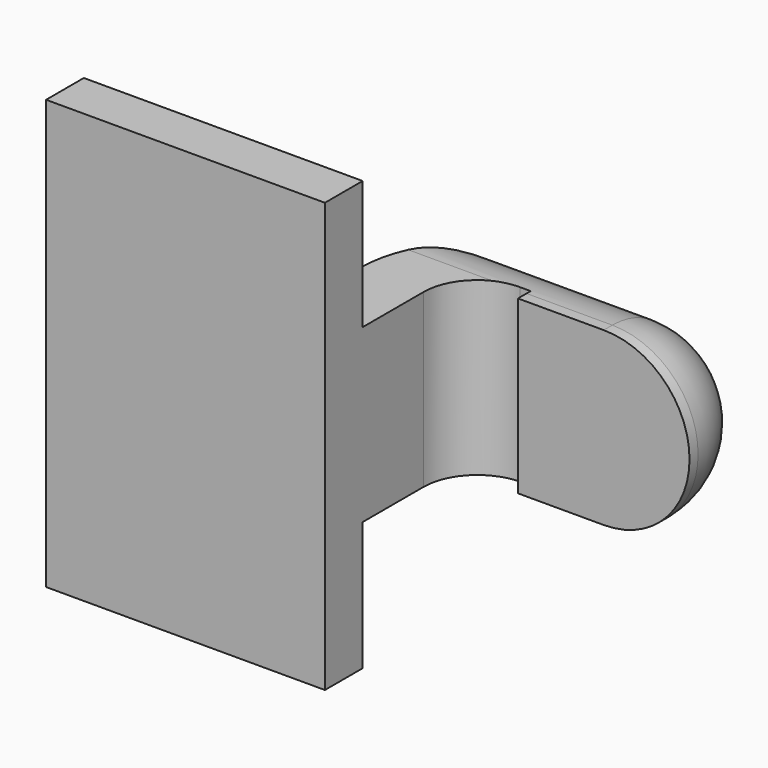
from build123d import *

# Parameters (mm, degrees)
F1_DEPTH    = 63.5
F0_W        = 25.4
F0_H        = 19.05
F0_H_2      = 4.7752
F0_H_3      = 4.7498
F2_DEPTH    = 25.4
F3_DEPTH    = 3.175
F5_T1_DEPTH = 88.9
F5_T4_ANGLE = 180
F6_SIZE     = 5.08


# Not quite as in the source:
# - a fillet or chamfer that OpenCascade refuses, or shapes differently, is made with other operations: its cross-section is extruded or revolved along the edge and cut away or added


with BuildPart() as f1:
    # F0 (on Top) → F1 (new body, symmetric)
    with BuildSketch(Plane.XY):
        Polygon((41.275, -9.525), (41.275, 9.525), (22.225, 9.525), (-41.275, 9.525), (-41.275, -9.525), align=None)
    extrude(amount=F1_DEPTH, both=True)

    # F0 (on Top) → F2 (join, symmetric)
    with BuildSketch(Plane.XY):
        with BuildLine():
            Line((22.225, 9.525), (41.275, 9.525))
            Line((41.275, 9.525), (41.275, 27.0002))
            ThreePointArc((41.275, 27.0002), (45.9246798487, 38.2255201513), (57.15, 42.8752))
            Line((57.15, 42.8752), (60.325, 42.8752))
            Line((60.325, 42.8752), (60.325, 61.9252))
            Line((60.325, 61.9252), (57.15, 61.9252))
            add(Edge.make_bspline(
                [(55.7653482616, 61.897740953), (56.229278457, 61.90719099), (56.6908681229, 61.9163212607), (57.15, 61.9252)],
                knots=[110.2179933389, 110.2179933389, 110.2179933389, 110.2179933389, 111.5045361635, 111.5045361635, 111.5045361635, 111.5045361635], degree=3))
            ThreePointArc((55.7653482616, 61.897740953), (31.9695056943, 51.2014051666), (22.225, 27.0002))
            Line((22.225, 27.0002), (22.225, 9.525))
        make_face()
        with Locations((73.025, 52.4002)):
            Rectangle(F0_W, F0_H)
        with Locations((73.025, 40.4876)):
            Rectangle(F0_W, F0_H_2)
        with Locations((73.025, 64.3001)):
            Rectangle(F0_W, F0_H_3)
    extrude(amount=F2_DEPTH, both=True)

    # F0 (on Top) → F3 (join, symmetric)
    with BuildSketch(Plane.XY):
        with BuildLine():
            Line((-41.275, 9.525), (22.225, 9.525))
            Line((22.225, 9.525), (22.225, 27.0002))
            ThreePointArc((22.225, 27.0002), (31.9695056943, 51.2014051666), (55.7653482616, 61.897740953))
            add(Edge.make_bspline(
                [(-41.275, 9.525), (-40.9022788448, 57.9317022513), (16.0204954638, 61.0881572363), (55.7653482616, 61.897740953)],
                knots=[0, 0, 0, 0, 110.2179933389, 110.2179933389, 110.2179933389, 110.2179933389], degree=3))
        make_face()
    extrude(amount=F3_DEPTH, both=True)

    # F0 (on Top) → F4 (revolve)
    with BuildSketch(Plane.XY):
        Polygon((85.725, 61.9252), (85.725, 42.8752), (85.725, 38.1), (111.125, 38.1), (111.125, 66.675), (85.725, 66.675), align=None)
    revolve(axis=Axis((85.725, 52.3875, 0), (0, 1, 0)))

    # F5: fillet of radius 25.4 on 1 edges, made by hand

    # F5_s2 → F5_t1 (cut)
    with BuildSketch(Plane.YZ.offset(-3.175)):
        with BuildLine():
            ThreePointArc((66.675, 0), (59.2355122421, -17.9605122421), (41.275, -25.4))
            Line((41.275, -25.4), (66.675, -25.4))
            Line((66.675, -25.4), (66.675, 0))
        make_face()
        with BuildLine():
            ThreePointArc((66.675, 0), (59.2355122421, 17.9605122421), (41.275, 25.4))
            Line((41.275, 25.4), (66.675, 25.4))
            Line((66.675, 25.4), (66.675, 0))
        make_face()
    extrude(amount=F5_T1_DEPTH, mode=Mode.SUBTRACT)

    # F5_s3 → F5_t4 (revolve, cut)
    with BuildSketch(Plane.YZ.offset(85.725)):
        with BuildLine():
            ThreePointArc((66.675, 0), (59.2355122421, -17.9605122421), (41.275, -25.4))
            Line((41.275, -25.4), (66.675, -25.4))
            Line((66.675, -25.4), (66.675, 0))
        make_face()
    revolve(axis=Axis((85.725, 66.675, 0), (0, -1, 0)), revolution_arc=F5_T4_ANGLE, mode=Mode.SUBTRACT)

    # F6
    f6_edges = [f1.edges().sort_by_distance(p)[0] for p in [
        (-9.525, 9.525, 3.175),
        (-9.525, 9.525, -3.175),
        (0, 9.525, -63.5),
        (41.275, 9.525, -44.45),
        (41.275, 9.525, 44.45),
        (0, 9.525, 63.5),
    ]]
    chamfer(f6_edges, length=F6_SIZE)


solid = f1.part
